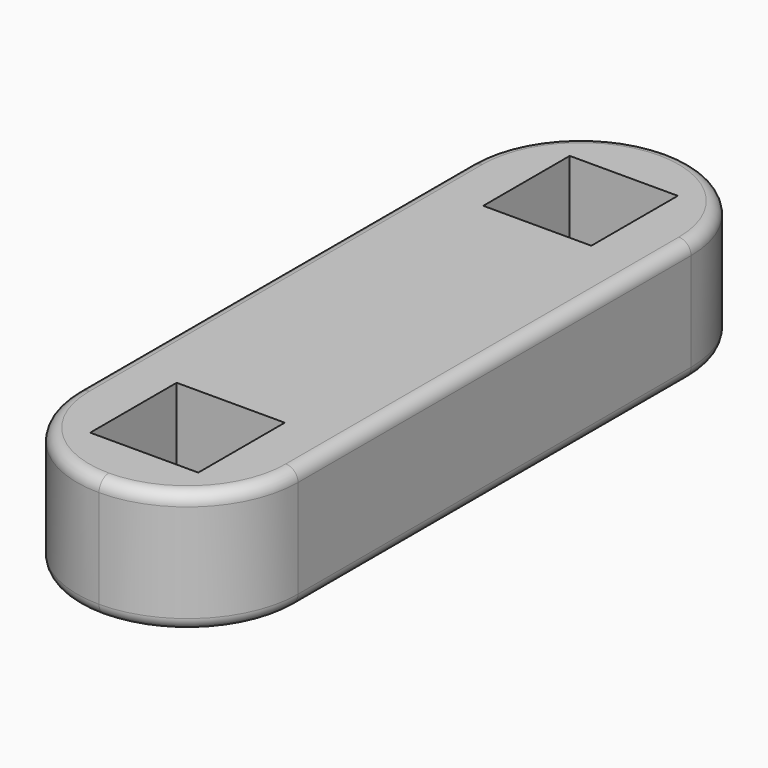
from build123d import *

# Parameters (mm, degrees)
F1_DEPTH = 5
F2_R     = 4.49999
F3_R     = 0.5


# Not quite as in the source:
# - a fillet or chamfer is up to 0.001 mm smaller than in the source, because OpenCascade refuses the exact size


with BuildPart() as f1:
    # F0 (on Top) → F1 (new body)
    with BuildSketch(Plane.XY):
        Polygon((4.5, -14.5), (4.5, 14.5), (0, 14.5), (-4.5, 14.5), (-4.5, -14.5), (0, -14.5), align=None)
        Polygon((2.2, -12.2), (0, -12.2), (-2.2, -12.2), (-2.2, -7.8), (2.2, -7.8), align=None, mode=Mode.SUBTRACT)
        Polygon((-2.2, 12.2), (0, 12.2), (2.2, 12.2), (2.2, 7.8), (-2.2, 7.8), align=None, mode=Mode.SUBTRACT)
    extrude(amount=F1_DEPTH)

    # F2 (radius 4.5 in the source; OpenCascade refuses exactly that, so slightly less here)
    f2_edges = [f1.edges().sort_by_distance(p)[0] for p in [
        (-4.5, 14.5, 2.5),
        (4.5, 14.5, 2.5),
        (4.5, -14.5, 2.5),
        (-4.5, -14.5, 2.5),
    ]]
    fillet(f2_edges, radius=F2_R)

    # F3
    f3_edges = [f1.edges().sort_by_distance(p)[0] for p in [
        (-4.5, 0, 5),
        (-4.5, 0, 0),
    ]]
    fillet(f3_edges, radius=F3_R)


solid = f1.part
